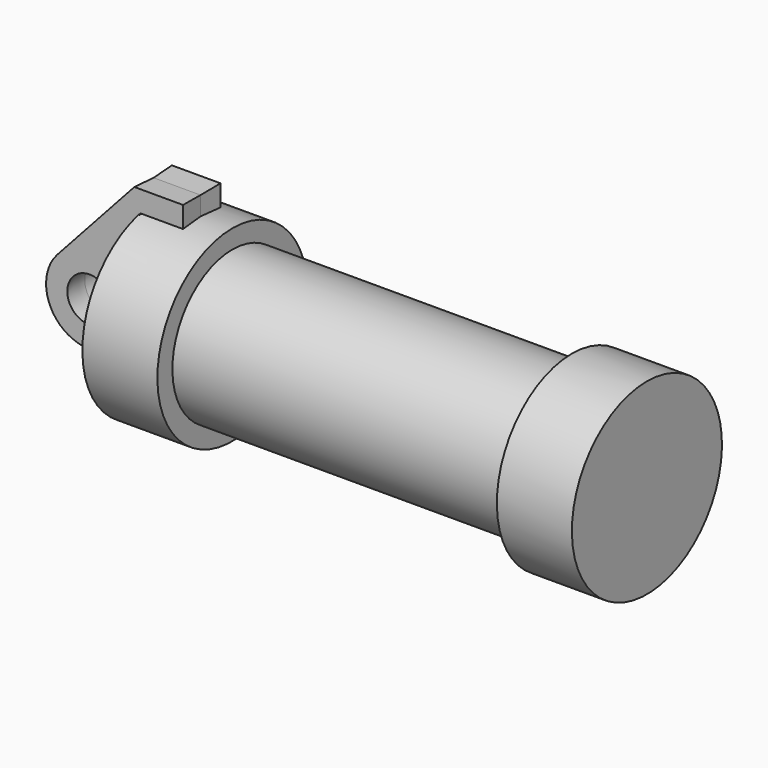
from build123d import *

# Parameters (mm, degrees)
F0_W     = 5.842
F0_H     = 12.7
F0_R     = 3.175
F2_DEPTH = 3.175
F2_TAPER = -3


# Not quite as in the source:
# - a feature names something its author has since deleted; it is built from what else it names


with BuildPart() as f1:
    # F0 (on Front) → F1 (revolve)
    with BuildSketch(Plane.XZ):
        with Locations((2.921, 6.35)):
            Rectangle(F0_W, F0_H)
        Polygon((5.842, 12.7), (5.842, 0), (66.294, 0), (66.294, 12.7), (56.134, 12.7), (56.134, 10.16), (10.16, 10.16), (10.16, 12.7), align=None)
    revolve(axis=Axis((33.147, 0, 0), (-1, 0, 0)))

    # F0 (on Front) → F2 (join, symmetric)
    with BuildSketch(Plane.XZ):
        with BuildLine():
            Line((-0.9398, 0), (0, 0))
            Line((0, 0), (0, 12.7))
            Line((0, 12.7), (5.842, 12.7))
            Line((5.842, 12.7), (5.842, 15.24))
            Line((5.842, 15.24), (-0.508, 15.24))
            Line((-0.508, 15.24), (-10.8806298187, 3.8475430269))
            ThreePointArc((-10.8806298187, 3.8475430269), (-4.5919612295, 5.3297205562), (-0.9398, 0))
        make_face()
        with BuildLine():
            ThreePointArc((-8.1826630726, -5.5069827884), (-3.1957909266, -4.5493385486), (-0.9398, 0))
            ThreePointArc((-0.9398, 0), (-4.5919612295, 5.3297205562), (-10.8806298187, 3.8475430269))
            ThreePointArc((-10.8806298187, 3.8475430269), (-12.1459778134, -1.5837270034), (-8.1826630726, -5.5069827884))
        make_face()
        with Locations((-6.6548, 0)):
            Circle(F0_R, mode=Mode.SUBTRACT)
        with BuildLine():
            Line((5.842, 0), (0, 0))
            Line((0, 0), (-0.9398, 0))
            ThreePointArc((-0.9398, 0), (-3.1957909266, -4.5493385486), (-8.1826630726, -5.5069827884))
            Line((-8.1826630726, -5.5069827884), (5.842, -9.398))
            Line((5.842, -9.398), (5.842, 0))
        make_face()
    extrude(amount=F2_DEPTH, both=True, taper=F2_TAPER)


solid = f1.part
